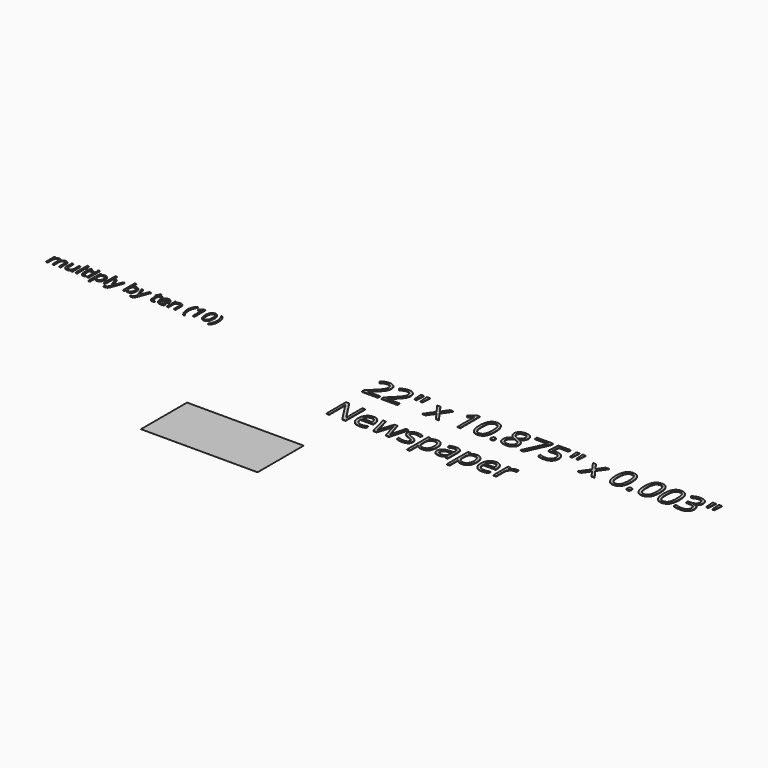
from build123d import *

# Parameters (mm, degrees)
F0_W         = 5588
F0_H         = 2762.25
F1_DEPTH     = 0.762
F2_TEXT_SIZE = 1631.6844357385
F3_DEPTH     = 25.4
F4_TEXT_SIZE = 916.0253736708
F5_DEPTH     = 25.4


# Not quite as in the source:
# - Text() gives the source's letters only with a copy of the font that has no kerning and outlines rounded to 1/6400 em; it was checked with that copy


with BuildPart() as f1:
    # F0 (on Top) → F1 (new body)
    with BuildSketch(Plane.XY):
        with Locations((2239.999294281, -5646.3504416842)):
            Rectangle(F0_W, F0_H)
    extrude(amount=F1_DEPTH)


with BuildPart() as f3:
    # F2 (on face) → F3 (new body)
    with BuildSketch(Plane.XY.offset(0.762)):
        with Locations((3937.9940032959, 490.2774095535)):
            Text('22" x 10.875" x 0.003"', F2_TEXT_SIZE, font='Open Sans', text_align=(TextAlign.LEFT, TextAlign.BOTTOM))
        with Locations((3937.9940032959, -1728.8134230508)):
            Text('Newspaper', F2_TEXT_SIZE, font='Open Sans', text_align=(TextAlign.LEFT, TextAlign.BOTTOM))
    extrude(amount=F3_DEPTH)


with BuildPart() as f5:
    # F4 (on Top) → F5 (new body)
    with BuildSketch(Plane.XY):
        with Locations((-11857.063293457, 1324.4953155518)):
            Text('multiply by ten (10)', F4_TEXT_SIZE, font='Open Sans', text_align=(TextAlign.LEFT, TextAlign.BOTTOM))
    extrude(amount=F5_DEPTH)


solid = Compound([f1.part, f3.part, f5.part])
